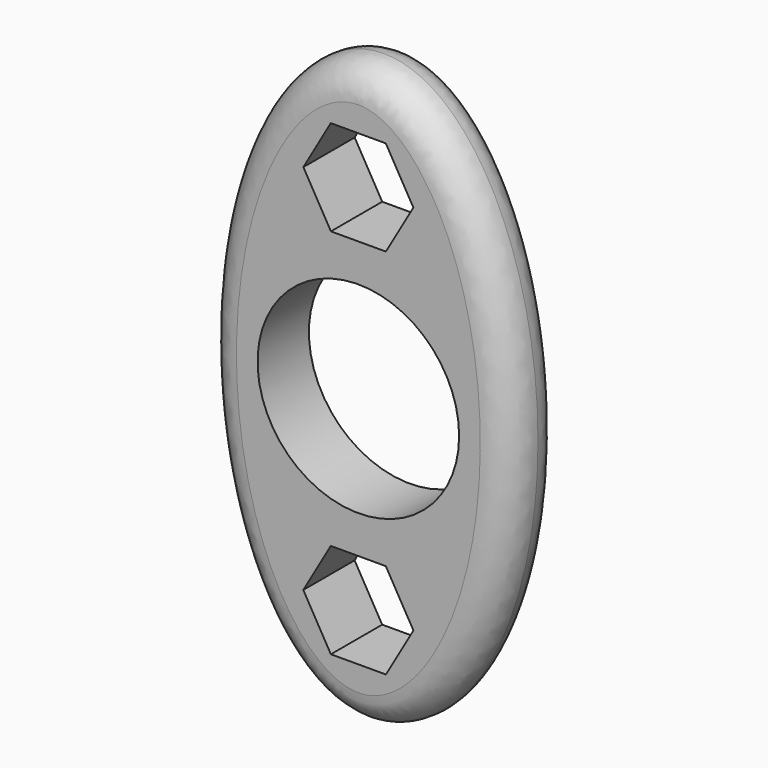
from build123d import *

# Parameters (mm, degrees)
F0_R     = 11
F1_DEPTH = 7
F2_R     = 3.4999


# Not quite as in the source:
# - a fillet or chamfer is up to 0.001 mm smaller than in the source, because OpenCascade refuses the exact size


with BuildPart() as f1:
    # F0 (on Front) → F1 (new body)
    with BuildSketch(Plane.XZ):
        with BuildLine():
            add(Edge.make_bspline(
                [(0, 31.75), (-29.1176115239, 31.75), (-14.558805762, -15.875), (0, -63.5), (14.558805762, -15.875), (29.1176115239, 31.75), (0, 31.75)],
                knots=[0, 0, 0, 2.0943951024, 2.0943951024, 4.1887902048, 4.1887902048, 6.2831853072, 6.2831853072, 6.2831853072], degree=2, weights=[1, 0.5, 1, 0.5, 1, 0.5, 1]))
        make_face()
        Polygon((2.9989406364, -15.1111775695), (6.0104428668, -20.3127475603), (3.0115022304, -25.5215699908), (-2.9989406364, -25.5288224305), (-6.0104428668, -20.3272524397), (-3.0115022304, -15.1184300092), align=None, mode=Mode.SUBTRACT)
        Circle(F0_R, mode=Mode.SUBTRACT)
        Polygon((2.9955036613, 25.5227137441), (6.0034341016, 20.3271746042), (3.0079304403, 15.1244608602), (-2.9955036613, 15.1172862559), (-6.0034341016, 20.3128253958), (-3.0079304403, 25.5155391398), align=None, mode=Mode.SUBTRACT)
    extrude(amount=F1_DEPTH)

    # F2 (radius 3.5 in the source; OpenCascade refuses exactly that, so slightly less here)
    f2_edges = [f1.edges().sort_by_distance(p)[0] for p in [
        (-2e-06, -7, -31.75),
        (-2e-06, 0, -31.75),
    ]]
    fillet(f2_edges, radius=F2_R)


solid = f1.part
